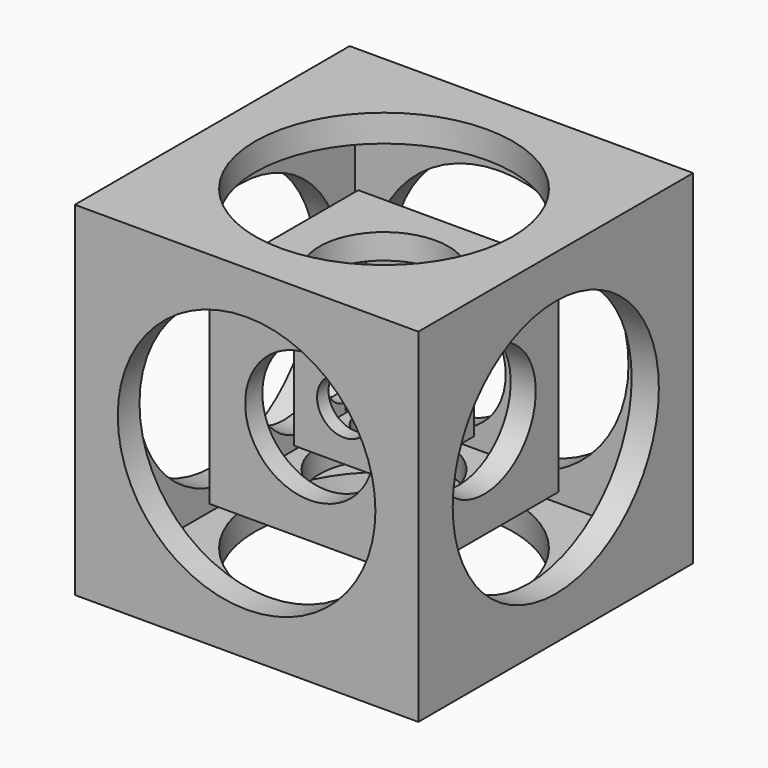
from build123d import *

# Parameters (mm, degrees)
F0_W      = 19.05
F0_H      = 19.05
F1_DEPTH  = 9.525
F2_W      = 44.45
F2_H      = 44.45
F2_W_2    = 31.75
F2_H_2    = 31.75
F3_DEPTH  = 22.225
F4_W      = 31.75
F4_H      = 31.75
F5_DEPTH  = 6.35
F6_W      = 31.75
F6_H      = 31.75
F7_DEPTH  = 6.35
F8_R      = 11.90625
F9_DEPTH  = 44.451
F10_R     = 11.90625
F11_DEPTH = 44.451
F12_R     = 11.90625
F13_DEPTH = 44.451
F14_W     = 88.9
F14_H     = 88.9
F14_W_2   = 66.675
F14_H_2   = 66.675
F15_DEPTH = 41.275
F16_W     = 66.675
F16_H     = 66.675
F17_DEPTH = 9.525
F18_W     = 66.675
F18_H     = 66.675
F19_DEPTH = 9.525
F20_R     = 28.575
F21_DEPTH = 82.551
F22_R     = 28.575
F23_DEPTH = 88.901
F24_R     = 28.575
F25_DEPTH = 88.901
F26_W     = 152.4
F26_H     = 152.4
F26_W_2   = 128.27
F26_H_2   = 128.27
F27_DEPTH = 76.2
F28_W     = 128.27
F28_H     = 128.27
F29_DEPTH = 12.065
F30_W     = 128.27
F30_H     = 128.27
F31_DEPTH = 12.065
F32_R     = 57.15
F33_DEPTH = 152.401
F34_R     = 57.15
F35_DEPTH = 152.401
F36_R     = 57.15
F37_DEPTH = 152.401


with BuildPart() as f1:
    # F0 (on Front) → F1 (new body, symmetric)
    with BuildSketch(Plane.XZ):
        Rectangle(F0_W, F0_H)
    extrude(amount=F1_DEPTH, both=True)


with BuildPart() as f3:
    # F2 (on Front) → F3 (new body, symmetric)
    with BuildSketch(Plane.XZ):
        Rectangle(F2_W, F2_H)
        Rectangle(F2_W_2, F2_H_2, mode=Mode.SUBTRACT)
    extrude(amount=F3_DEPTH, both=True)

    # F4 (on face) → F5 (join)
    with BuildSketch(Plane.XZ.offset(22.225)):
        Rectangle(F4_W, F4_H)
    extrude(amount=-F5_DEPTH)

    # F6 (on face) → F7 (join)
    with BuildSketch(Plane(origin=(0, 22.225, 0), x_dir=(-1, 0, 0), z_dir=(0, 1, 0))):
        Rectangle(F6_W, F6_H)
    extrude(amount=-F7_DEPTH)

    # F8 (on face) → F9 (cut, through all)
    with BuildSketch(Plane(origin=(0, 22.225, 0), x_dir=(-1, 0, 0), z_dir=(0, 1, 0))):
        Circle(F8_R)
    extrude(amount=-F9_DEPTH, mode=Mode.SUBTRACT)

    # F10 (on face) → F11 (cut, through all)
    with BuildSketch(Plane.YZ.offset(22.225)):
        Circle(F10_R)
    extrude(amount=-F11_DEPTH, mode=Mode.SUBTRACT)

    # F12 (on face) → F13 (cut, through all)
    with BuildSketch(Plane(origin=(0, 0, -22.225), x_dir=(1, 0, 0), z_dir=(0, 0, -1))):
        Circle(F12_R)
    extrude(amount=-F13_DEPTH, mode=Mode.SUBTRACT)


with BuildPart() as f15:
    # F14 (on Front) → F15 (new body, symmetric)
    with BuildSketch(Plane.XZ):
        Rectangle(F14_W, F14_H)
        Rectangle(F14_W_2, F14_H_2, mode=Mode.SUBTRACT)
    extrude(amount=F15_DEPTH, both=True)

    # F16 (on face) → F17 (join)
    with BuildSketch(Plane(origin=(0, 41.275, 0), x_dir=(-1, 0, 0), z_dir=(0, 1, 0))):
        Rectangle(F16_W, F16_H)
    extrude(amount=-F17_DEPTH)

    # F18 (on face) → F19 (join)
    with BuildSketch(Plane.XZ.offset(41.275)):
        Rectangle(F18_W, F18_H)
    extrude(amount=-F19_DEPTH)

    # F20 (on face) → F21 (cut, through all)
    with BuildSketch(Plane.XZ.offset(41.275)):
        Circle(F20_R)
    extrude(amount=-F21_DEPTH, mode=Mode.SUBTRACT)

    # F22 (on face) → F23 (cut, through all)
    with BuildSketch(Plane(origin=(-44.45, 0, 0), x_dir=(0, -1, 0), z_dir=(-1, 0, 0))):
        Circle(F22_R)
    extrude(amount=-F23_DEPTH, mode=Mode.SUBTRACT)

    # F24 (on face) → F25 (cut, through all)
    with BuildSketch(Plane.XY.offset(44.45)):
        Circle(F24_R)
    extrude(amount=-F25_DEPTH, mode=Mode.SUBTRACT)


with BuildPart() as f27:
    # F26 (on Front) → F27 (new body, symmetric)
    with BuildSketch(Plane.XZ):
        Rectangle(F26_W, F26_H)
        Rectangle(F26_W_2, F26_H_2, mode=Mode.SUBTRACT)
    extrude(amount=F27_DEPTH, both=True)

    # F28 (on face) → F29 (join)
    with BuildSketch(Plane.XZ.offset(76.2)):
        Rectangle(F28_W, F28_H)
    extrude(amount=-F29_DEPTH)

    # F30 (on face) → F31 (join)
    with BuildSketch(Plane(origin=(0, 76.2, 0), x_dir=(-1, 0, 0), z_dir=(0, 1, 0))):
        Rectangle(F30_W, F30_H)
    extrude(amount=-F31_DEPTH)

    # F32 (on face) → F33 (cut, through all)
    with BuildSketch(Plane.XZ.offset(76.2)):
        Circle(F32_R)
    extrude(amount=-F33_DEPTH, mode=Mode.SUBTRACT)

    # F34 (on face) → F35 (cut, through all)
    with BuildSketch(Plane(origin=(-76.2, 0, 0), x_dir=(0, -1, 0), z_dir=(-1, 0, 0))):
        Circle(F34_R)
    extrude(amount=-F35_DEPTH, mode=Mode.SUBTRACT)

    # F36 (on face) → F37 (cut, through all)
    with BuildSketch(Plane.XY.offset(76.2)):
        Circle(F36_R)
    extrude(amount=-F37_DEPTH, mode=Mode.SUBTRACT)


solid = Compound([f1.part, f3.part, f15.part, f27.part])
